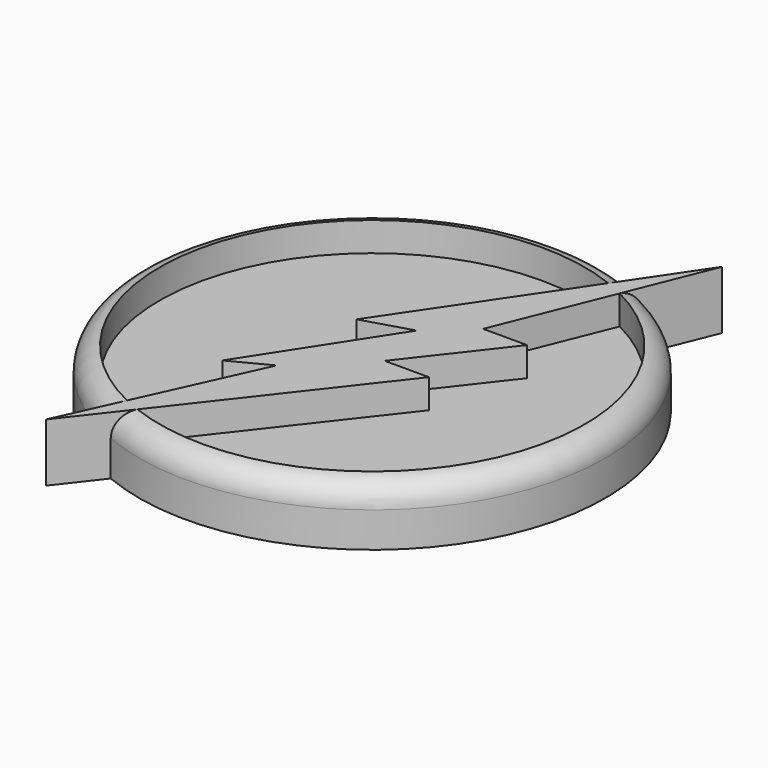
from build123d import *

# Parameters (mm, degrees)
F0_R     = 46.303997109
F1_DEPTH = 6.35
F0_R_2   = 50.7773250867
F2_DEPTH = 12.7
F5_DEPTH = 6.35
F6_DEPTH = 12.7


# Not quite as in the source:
# - a fillet or chamfer that OpenCascade refuses, or shapes differently, is made with other operations: its cross-section is extruded or revolved along the edge and cut away or added


with BuildPart() as f1:
    # F0 (on Top) → F1 (new body)
    with BuildSketch(Plane.XY):
        Circle(F0_R)
    extrude(amount=F1_DEPTH)

    # F0 (on Top) → F2 (join)
    with BuildSketch(Plane.XY):
        Circle(F0_R_2)
        Circle(F0_R, mode=Mode.SUBTRACT)
    extrude(amount=F2_DEPTH)

    # F3: fillet of radius 5.08 on 1 edges, made by hand

    # F3_s1 → F3_t2 (revolve, cut)
    with BuildSketch(Plane.XZ):
        with BuildLine():
            ThreePointArc((50.7773250867, 7.6563555778), (49.4978706971, 11.0271497073), (46.303997109, 12.7))
            Line((46.303997109, 12.7), (46.3161305494, 12.8008728884))
            ThreePointArc((46.3161305494, 12.8008728884), (48.5406610978, 12.8016), (50.7773250867, 12.8016))
            Line((50.7773250867, 12.8016), (50.8789250867, 12.7))
            Line((50.8789250867, 12.7), (50.8789250867, 7.6563555778))
            Line((50.8789250867, 7.6563555778), (50.7773250867, 7.6563555778))
        make_face()
    revolve(axis=Axis((0, 0, 12.7), (0, 0, 1)), mode=Mode.SUBTRACT)

    # F4 (on face) → F5 (join)
    with BuildSketch(Plane.XY.offset(6.35)):
        Polygon((-8.1779062748, -15.8028278183), (-26.3735784938, -55.8334334653), (14.7386826575, -3.0078946147), (5.1134219393, -3.0078946147), (20.4086864271, 16.6451374931), (10.8284205198, 16.6451374931), (28.2742083073, 59.8571076989), (-8.1779062748, 5.9409798123), (2.4016224779, 9.0941041708), (-16.5434218943, -20.15289478), align=None)
    extrude(amount=F5_DEPTH)

    # F6 (add): a face of the model
    f6_faces = [f1.faces().sort_by_distance(p)[0] for p in [
        (2.0188421937, 0.3767409736, 12.7),
    ]]
    extrude(f6_faces, amount=-F6_DEPTH)


solid = f1.part
